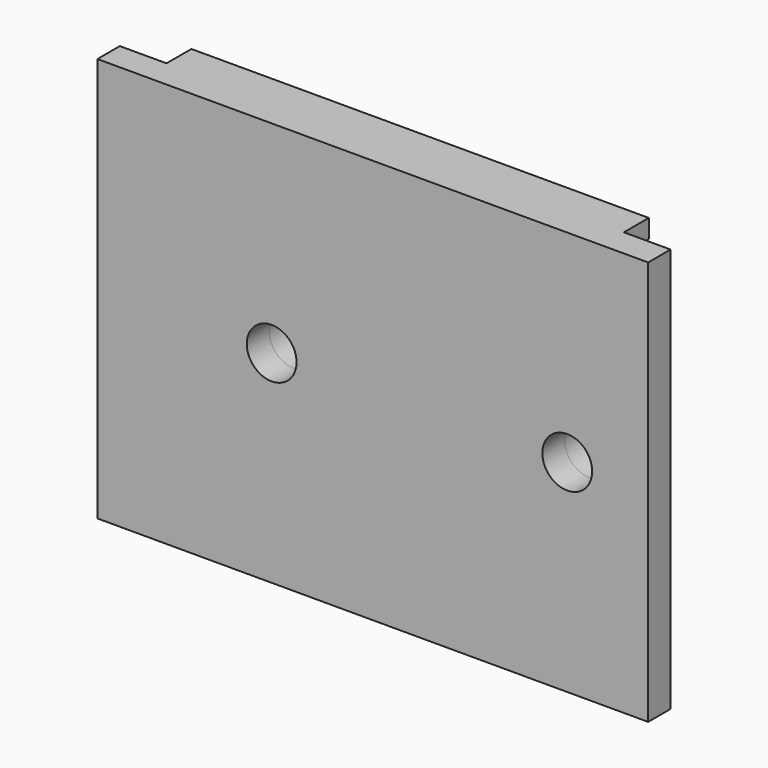
from build123d import *

# Parameters (mm, degrees)
F0_R     = 3
F0_W     = 29.4
F0_H     = 1.2
F0_R_2   = 1.6
F1_DEPTH = 1.8
F2_DEPTH = 2


# Not quite as in the source:
# - a feature names something its author has since deleted; it is built from what else it names


with BuildPart() as f1:
    # F0 (on Front) → F1 (new body)
    with BuildSketch(Plane.XZ):
        Polygon((-14.7, 13), (-17.7, 13), (-17.7, -13), (-14.7, -13), (-14.7, -11.8), (14.7, -11.8), (14.7, -13), (17.7, -13), (17.7, 13), (14.7, 13), (14.7, 11.8), (-14.7, 11.8), align=None)
        with Locations((-6.5, 0)):
            Circle(F0_R, mode=Mode.SUBTRACT)
        with Locations((12.5, 0)):
            Circle(F0_R, mode=Mode.SUBTRACT)
        with Locations((0, 12.4)):
            Rectangle(F0_W, F0_H)
        with Locations((0, -12.4)):
            Rectangle(F0_W, F0_H)
        with Locations((-6.5, 0)):
            Circle(F0_R)
        with Locations((-6.5, 0)):
            Circle(F0_R_2, mode=Mode.SUBTRACT)
        with Locations((12.5, 0)):
            Circle(F0_R)
        with Locations((12.5, 0)):
            Circle(F0_R_2, mode=Mode.SUBTRACT)
    extrude(amount=F1_DEPTH)

    # F0 (on Front) → F2 (join)
    with BuildSketch(Plane.XZ):
        with Locations((12.5, 0)):
            Circle(F0_R)
        with Locations((12.5, 0)):
            Circle(F0_R_2, mode=Mode.SUBTRACT)
        with Locations((-6.5, 0)):
            Circle(F0_R)
        with Locations((-6.5, 0)):
            Circle(F0_R_2, mode=Mode.SUBTRACT)
        with Locations((0, 12.4)):
            Rectangle(F0_W, F0_H)
        with Locations((0, -12.4)):
            Rectangle(F0_W, F0_H)
    extrude(amount=-F2_DEPTH)


solid = f1.part
